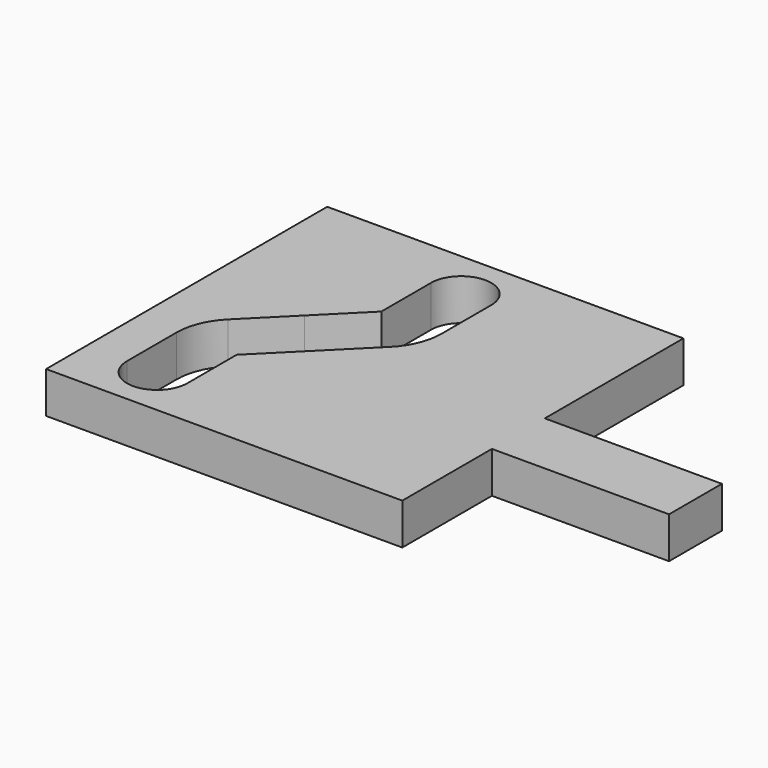
from build123d import *

# Parameters (mm, degrees)
F1_DEPTH = 8.89


# Not quite as in the source:
# - ends of sketch curves that miss each other by under 0.0002 mm in the source are joined


with BuildPart() as f1:
    # F0 (on Top) → F1 (new body)
    with BuildSketch(Plane.XY):
        Polygon((-80.7234341223, 10.5582008122), (-130.004342081, 10.5582008122), (-157.3788927812, 10.5582008122), (-157.3788927812, -26.3808563827), (-157.3788927812, -65.0632401945), (-80.7234341223, -65.0632401945), (-80.7234341223, -40.955274603), (-42.608632099, -40.955274603), (-42.608632099, -33.843274603), (-42.608632099, -26.731274603), (-80.7234341223, -26.731274603), align=None)
        with BuildLine():
            Line((-135.6170021567, -22.6889609682), (-130.004342081, -17.0763008925))
            Line((-130.004342081, -17.0763008925), (-126.4574508613, -13.5294096728))
            Line((-126.4574508613, -13.5294096728), (-126.4574508613, -0.1613896728))
            ThreePointArc((-126.4574508613, -0.1613896728), (-119.9804508613, 6.3156103272), (-113.5034508613, -0.1613896728))
            Line((-113.5034508613, -0.1613896728), (-113.5034508613, -13.5294096728))
            ThreePointArc((-113.5034508613, -13.5294096728), (-114.4895153971, -18.4866908556), (-117.2975896178, -22.6892709163))
            Line((-117.2975896178, -22.6892709163), (-126.4526293546, -31.8443106531))
            Line((-126.4526293546, -31.8443106531), (-135.6124905981, -41.0041718966))
            Line((-135.6124905981, -41.0041718966), (-135.6124905981, -54.3040225299))
            ThreePointArc((-135.6124905981, -54.3040225299), (-142.089490459, -60.7810223908), (-148.56649032, -54.3040225299))
            Line((-148.56649032, -54.3040225299), (-148.56649032, -41.0041716185))
            ThreePointArc((-148.56649032, -41.0041716185), (-147.5816463153, -36.0498380851), (-144.7768622884, -31.8488233223))
            Line((-144.7768622884, -31.8488233223), (-144.7723515635, -31.844310375))
            Line((-144.7723515635, -31.844310375), (-135.6173121048, -22.6892709163))
            Line((-135.6173121048, -22.6892709163), (-135.6170021567, -22.6889609682))
        make_face(mode=Mode.SUBTRACT)
    extrude(amount=F1_DEPTH)


solid = f1.part
